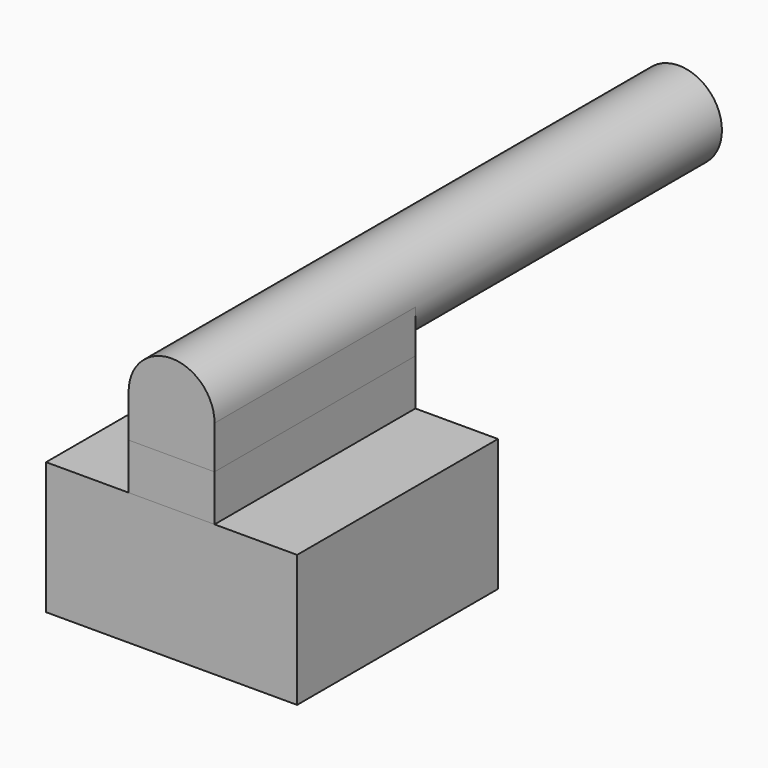
from build123d import *

# Parameters (mm, degrees)
F0_W     = 94.996
F0_H     = 49.9872
F1_DEPTH = 94.996
F2_W     = 32.512
F2_H     = 17.5006
F3_DEPTH = 94.996
F4_R     = 16.256
F5_DEPTH = 240.0046
F6_W     = 32.512
F6_H     = 16.256
F7_DEPTH = 94.996


with BuildPart() as f1:
    # F0 (on Front) → F1 (new body)
    with BuildSketch(Plane.XZ):
        with Locations((2.7489867061, -17.7890766389)):
            Rectangle(F0_W, F0_H)
    extrude(amount=F1_DEPTH)


with BuildPart() as f3:
    # F2 (on face) → F3 (new body)
    with BuildSketch(Plane.XZ.offset(94.996)):
        with Locations((2.7489867061, 15.9548233611)):
            Rectangle(F2_W, F2_H)
    extrude(amount=-F3_DEPTH)


with BuildPart() as f5:
    # F4 (on face) → F5 (new body)
    with BuildSketch(Plane.XZ.offset(94.996)):
        with Locations((2.7489867061, 40.9611233611)):
            Circle(F4_R)
    extrude(amount=-F5_DEPTH)

    # F6 (on face) → F7 (join)
    with BuildSketch(Plane.XZ.offset(94.996)):
        with Locations((2.7489867061, 32.8331233611)):
            Rectangle(F6_W, F6_H)
    extrude(amount=-F7_DEPTH)


solid = Compound([f1.part, f3.part, f5.part])
